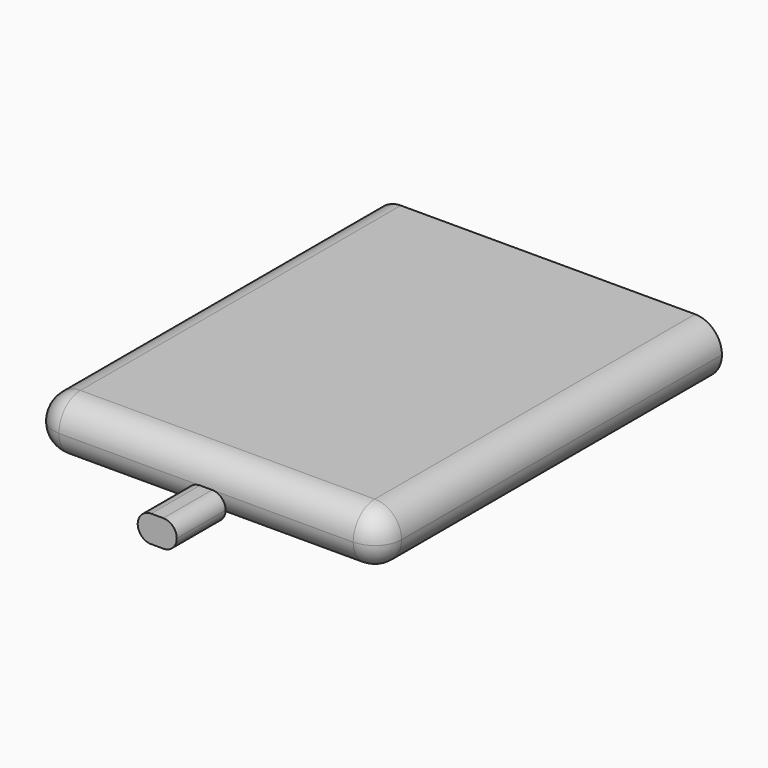
from build123d import *

# Parameters (mm, degrees)
F1_DEPTH = 88.9
F3_R     = 5.58799
F4_DEPTH = 12.7


# Not quite as in the source:
# - a fillet or chamfer is up to 0.001 mm smaller than in the source, because OpenCascade refuses the exact size


with BuildPart() as f1:
    # F0 (on Front) → F1 (new body)
    with BuildSketch(Plane.XZ):
        with BuildLine():
            ThreePointArc((-25.019, -5.588), (-26.6556873013, -1.6366873121), (-30.6069999848, 0))
            ThreePointArc((-30.6069999848, 0), (-34.5583126879, -1.6366873013), (-36.195, -5.588))
            ThreePointArc((-36.195, -5.588), (-34.5583126933, -9.5393126933), (-30.607, -11.176))
            ThreePointArc((-30.607, -11.176), (-26.6556873067, -9.5393126933), (-25.019, -5.588))
        make_face()
        with BuildLine():
            Line((0, -11.176), (0, 0))
            Line((0, 0), (-30.6069999848, 0))
            ThreePointArc((-30.6069999848, 0), (-26.6556873013, -1.6366873121), (-25.019, -5.588))
            ThreePointArc((-25.019, -5.588), (-26.6556873067, -9.5393126933), (-30.607, -11.176))
            Line((-30.607, -11.176), (0, -11.176))
        make_face()
        with BuildLine():
            Line((30.607, 0), (0, 0))
            Line((0, 0), (0, -11.176))
            Line((0, -11.176), (30.607, -11.176))
            ThreePointArc((30.607, -11.176), (25.019, -5.588), (30.607, 0))
        make_face()
        with BuildLine():
            ThreePointArc((36.195, -5.588), (34.5583126933, -1.6366873067), (30.607, 0))
            ThreePointArc((30.607, 0), (25.019, -5.588), (30.607, -11.176))
            ThreePointArc((30.607, -11.176), (34.5583126933, -9.5393126933), (36.195, -5.588))
        make_face()
    extrude(amount=F1_DEPTH)

    # F3 (radius 5.588 in the source; OpenCascade refuses exactly that, so slightly less here)
    f3_edges = [f1.edges().sort_by_distance(p)[0] for p in [
        (0, -88.9, 0),
        (-36.195, -88.9, -5.588),
        (36.195, -88.9, -5.588),
    ]]
    fillet(f3_edges, radius=F3_R)


with BuildPart() as f4:
    # F2 (on face) → F4 (new body)
    with BuildSketch(Plane.XZ.offset(88.9)):
        with BuildLine():
            ThreePointArc((0, -5.8933184213), (-0.6169074839, -5.6654017291), (-1.27, -5.588))
            ThreePointArc((-1.27, -5.588), (-3.2456563466, -6.4063436534), (-4.064, -8.382))
            Line((-4.064, -8.382), (-1.524, -8.382))
            ThreePointArc((-1.524, -8.382), (-1.112731206, -6.9228810878), (0, -5.8933184213))
        make_face()
        with BuildLine():
            Line((0, -5.588), (-1.27, -5.588))
            ThreePointArc((-1.27, -5.588), (-0.6169074839, -5.6654017291), (0, -5.8933184213))
            Line((0, -5.8933184213), (0, -5.588))
        make_face()
        with BuildLine():
            Line((1.27, -5.588), (0, -5.588))
            Line((0, -5.588), (0, -5.8933184213))
            ThreePointArc((0, -5.8933184213), (0.6169074839, -5.6654017291), (1.27, -5.588))
        make_face()
        with BuildLine():
            Line((-1.524, -8.382), (-4.064, -8.382))
            ThreePointArc((-4.064, -8.382), (-3.2456563466, -10.3576563466), (-1.27, -11.176))
            ThreePointArc((-1.27, -11.176), (-0.6169074839, -11.0985982709), (0, -10.8706815787))
            ThreePointArc((0, -10.8706815787), (-1.112731206, -9.8411189122), (-1.524, -8.382))
        make_face()
        with BuildLine():
            ThreePointArc((1.524, -8.382), (1.112731206, -6.9228810878), (0, -5.8933184213))
            Line((0, -5.8933184213), (0, -8.382))
            Line((0, -8.382), (1.27, -8.382))
            Line((1.27, -8.382), (1.524, -8.382))
        make_face()
        with BuildLine():
            ThreePointArc((1.27, -5.588), (0.6169074839, -5.6654017291), (0, -5.8933184213))
            ThreePointArc((0, -5.8933184213), (1.112731206, -6.9228810878), (1.524, -8.382))
            Line((1.524, -8.382), (4.064, -8.382))
            ThreePointArc((4.064, -8.382), (3.2456563466, -6.4063436534), (1.27, -5.588))
        make_face()
        with BuildLine():
            Line((0, -8.382), (0, -5.8933184213))
            ThreePointArc((0, -5.8933184213), (-1.112731206, -6.9228810878), (-1.524, -8.382))
            Line((-1.524, -8.382), (-1.27, -8.382))
            Line((-1.27, -8.382), (0, -8.382))
        make_face()
        with BuildLine():
            ThreePointArc((0, -10.8706815787), (-0.6169074839, -11.0985982709), (-1.27, -11.176))
            Line((-1.27, -11.176), (0, -11.176))
            Line((0, -11.176), (0, -10.8706815787))
        make_face()
        with BuildLine():
            Line((-1.27, -8.382), (-1.524, -8.382))
            ThreePointArc((-1.524, -8.382), (-1.112731206, -9.8411189122), (0, -10.8706815787))
            Line((0, -10.8706815787), (0, -8.382))
            Line((0, -8.382), (-1.27, -8.382))
        make_face()
        with BuildLine():
            Line((1.27, -8.382), (0, -8.382))
            Line((0, -8.382), (0, -10.8706815787))
            ThreePointArc((0, -10.8706815787), (1.112731206, -9.8411189122), (1.524, -8.382))
            Line((1.524, -8.382), (1.27, -8.382))
        make_face()
        with BuildLine():
            Line((4.064, -8.382), (1.524, -8.382))
            ThreePointArc((1.524, -8.382), (1.112731206, -9.8411189122), (0, -10.8706815787))
            ThreePointArc((0, -10.8706815787), (0.6169074839, -11.0985982709), (1.27, -11.176))
            ThreePointArc((1.27, -11.176), (3.2456563466, -10.3576563466), (4.064, -8.382))
        make_face()
        with BuildLine():
            ThreePointArc((1.27, -11.176), (0.6169074839, -11.0985982709), (0, -10.8706815787))
            Line((0, -10.8706815787), (0, -11.176))
            Line((0, -11.176), (1.27, -11.176))
        make_face()
    extrude(amount=F4_DEPTH)


solid = Compound([f1.part, f4.part])
